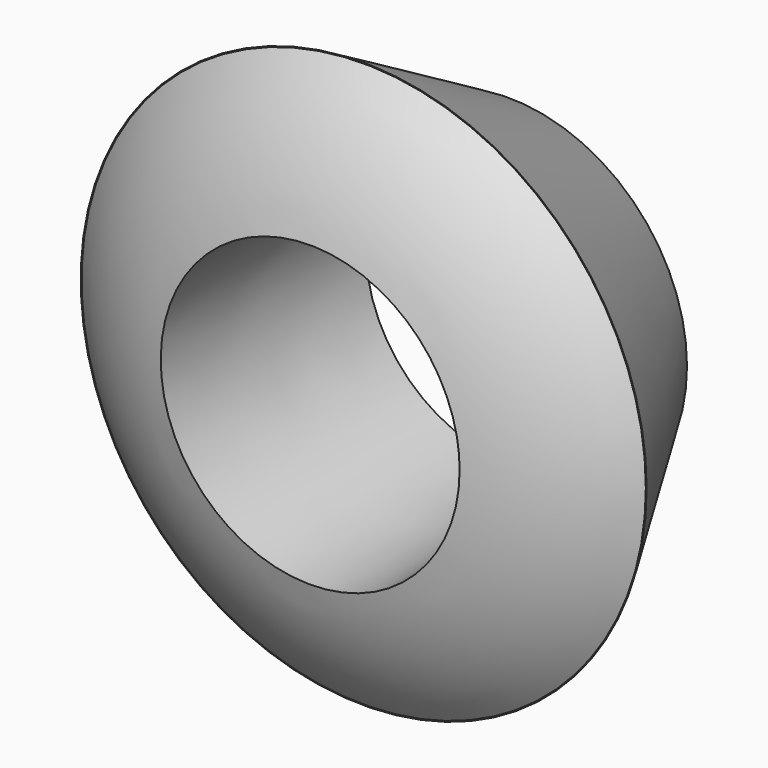
from build123d import *

# Parameters (mm, degrees)
F0_R           = 25
F1_DEPTH       = 25.4
F1_TAPER       = -30
F3_R           = 39.5485289591
F4_DEPTH       = 10.16
F6_R           = 20.0377303014
F7_DEPTH       = 35.5610001
F7_TAPER       = -1.5
F8_R           = 1.8145667082
F9_DEPTH       = 12.7
F9_DEPTH_BACK  = 25.4
F8_R_2         = 1.8161
F10_DEPTH      = 12.7
F10_DEPTH_BACK = 12.7
F11_DEPTH      = 12.7


# Not quite as in the source:
# - a fillet or chamfer that OpenCascade refuses, or shapes differently, is made with other operations: its cross-section is extruded or revolved along the edge and cut away or added


with BuildPart() as f1:
    # F0 (on Front) → F1 (new body)
    with BuildSketch(Plane.XZ):
        Circle(F0_R)
    extrude(amount=F1_DEPTH, taper=F1_TAPER)

    # F3 (on offset) → F4 (join)
    with BuildSketch(Plane.XZ.offset(25.4)):
        Circle(F3_R)
    extrude(amount=F4_DEPTH)

    # F5: fillet of radius 39.497 on 1 edges, made by hand

    # F5_s1 → F5_t2 (revolve, cut)
    with BuildSketch(Plane.XY):
        with BuildLine():
            ThreePointArc((39.5485289591, -25.4), (27.2681504962, -32.9326114571), (13.1032375067, -35.56))
            Line((13.1032375067, -35.56), (13.1032375067, -36.34994))
            Line((13.1032375067, -36.34994), (39.5485289591, -36.34994))
            Line((39.5485289591, -36.34994), (40.3384689591, -35.56))
            ThreePointArc((40.3384689591, -35.56), (40.3384689591, -30.48), (40.0774347881, -25.98674))
            Line((40.0774347881, -25.98674), (39.5485289591, -25.4))
        make_face()
    revolve(axis=Axis((0, -35.56, 0), (0, -1, 0)), mode=Mode.SUBTRACT)

    # F6 (on Front) → F7 (cut, through all)
    with BuildSketch(Plane.XZ):
        Circle(F6_R)
    extrude(amount=F7_DEPTH, taper=F7_TAPER, mode=Mode.SUBTRACT)

    # F8 (on Front) → F9 (cut, two sides)
    with BuildSketch(Plane.XZ) as f9_sk:
        with Locations((0, 22.6314)):
            Circle(F8_R)
    extrude(amount=F9_DEPTH, mode=Mode.SUBTRACT)
    extrude(f9_sk.sketch, amount=-F9_DEPTH_BACK, mode=Mode.SUBTRACT)

    # F8 (on Front) → F10 (cut, two sides)
    with BuildSketch(Plane.XZ) as f10_sk:
        with Locations((22.6314, 0)):
            Circle(F8_R_2)
    extrude(amount=-F10_DEPTH, mode=Mode.SUBTRACT)
    extrude(f10_sk.sketch, amount=F10_DEPTH_BACK, mode=Mode.SUBTRACT)

    # F8 (on Front) → F11 (cut)
    with BuildSketch(Plane.XZ):
        with Locations((0, 22.6314)):
            Circle(F8_R)
        with Locations((22.6314, 0)):
            Circle(F8_R_2)
        with Locations((0, -22.6314)):
            Circle(F8_R_2)
        with Locations((-22.6314, 0)):
            Circle(F8_R_2)
    extrude(amount=F11_DEPTH, mode=Mode.SUBTRACT)


solid = f1.part
